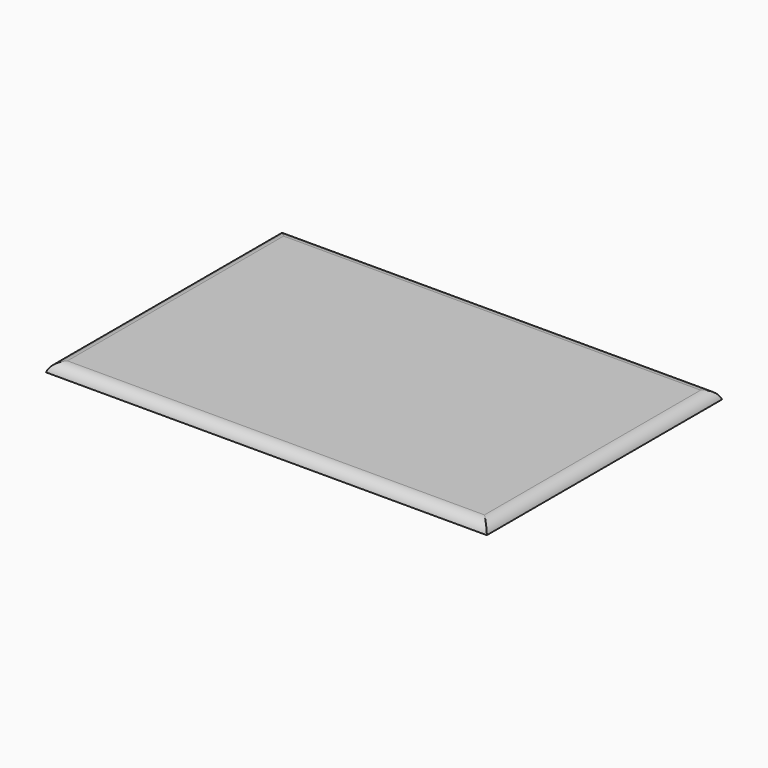
from build123d import *

# Parameters (mm, degrees)
F0_W        = 914.4
F0_H        = 609.6
F1_DEPTH    = 19.05
F2_T1_DEPTH = 732.5672212421
F2_T3_DEPTH = 1037.3672212421


# Not quite as in the source:
# - a fillet or chamfer that OpenCascade refuses, or shapes differently, is made with other operations: its cross-section is extruded or revolved along the edge and cut away or added


with BuildPart() as f1:
    # F0 (on Top) → F1 (new body)
    with BuildSketch(Plane.XY):
        with Locations((-457.2, 142.6232497496)):
            Rectangle(F0_W, F0_H)
    extrude(amount=F1_DEPTH)

    # F2: fillet of radius 25.4 on 4 edges, made by hand

    # F2_s2 → F2_t1 (cut)
    with BuildSketch(Plane.XZ.offset(-508.9068603707)):
        with BuildLine():
            ThreePointArc((0, 0), (-9.0391843817, 13.7304631421), (-24.5934442484, 19.05))
            Line((-24.5934442484, 19.05), (0, 19.05))
            Line((0, 19.05), (0, 0))
        make_face()
        with BuildLine():
            ThreePointArc((-914.4, 0), (-905.3608156183, 13.7304631421), (-889.8065557516, 19.05))
            Line((-889.8065557516, 19.05), (-914.4, 19.05))
            Line((-914.4, 19.05), (-914.4, 0))
        make_face()
    extrude(amount=F2_T1_DEPTH, mode=Mode.SUBTRACT)

    # F2_s4 → F2_t3 (cut)
    with BuildSketch(Plane.YZ.offset(-975.883610621)):
        with BuildLine():
            ThreePointArc((-162.1767502504, 0), (-153.1375658686, 13.7304631421), (-137.583306002, 19.05))
            Line((-137.583306002, 19.05), (-162.1767502504, 19.05))
            Line((-162.1767502504, 19.05), (-162.1767502504, 0))
        make_face()
        with BuildLine():
            ThreePointArc((447.4232497496, 0), (438.3840653679, 13.7304631421), (422.8298055012, 19.05))
            Line((422.8298055012, 19.05), (447.4232497496, 19.05))
            Line((447.4232497496, 19.05), (447.4232497496, 0))
        make_face()
    extrude(amount=F2_T3_DEPTH, mode=Mode.SUBTRACT)


solid = f1.part
